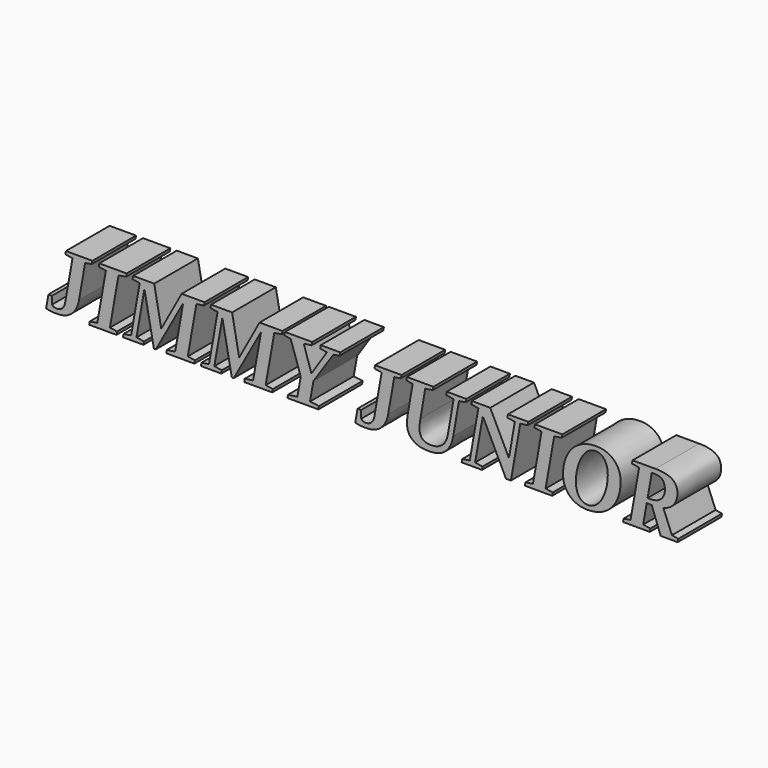
from build123d import *

# Parameters (mm, degrees)
F0_TEXT_SIZE = 40.74863391
F1_DEPTH     = 25.4


# Not quite as in the source:
# - Text() gives the source's letters only with a copy of the font that has no kerning and outlines rounded to 1/6400 em; it was checked with that copy


with BuildPart() as f1:
    # F0 (on Front) → F1 (new body)
    with BuildSketch(Plane.XZ):
        with Locations((-54.5404776931, 7.3347566649)):
            Text('JIMMY JUNIOR', F0_TEXT_SIZE, font='Tinos', font_style=FontStyle.BOLDITALIC, text_align=(TextAlign.LEFT, TextAlign.BOTTOM))
    extrude(amount=F1_DEPTH)


solid = f1.part
